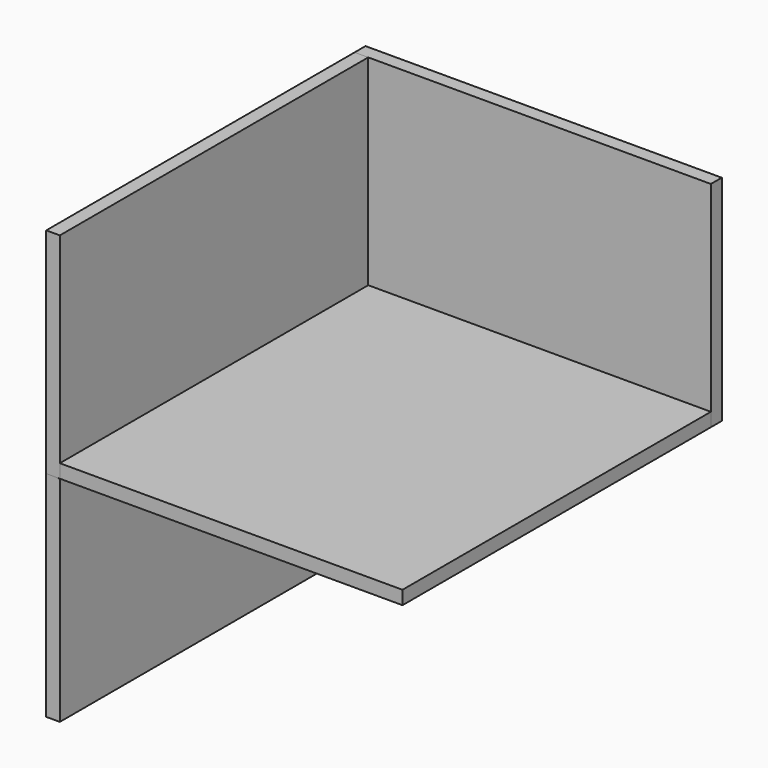
from build123d import *

# Parameters (mm, degrees)
F0_W           = 83.175
F0_H           = 50
F1_DEPTH       = 3.175
F2_W           = 3.175
F2_H           = 50
F3_DEPTH       = 90
F4_W           = 3.175
F4_H           = 50
F5_DEPTH       = 80
F6_W           = 80
F6_H           = 3.175
F7_DEPTH       = 90
F8_W           = 80
F8_H           = 3.175
F9_DEPTH       = 80
F10_W          = 3.175
F10_H          = 50
F11_DEPTH      = 90
F11_DEPTH_BACK = 3.175
F12_R          = 2.5
F13_DEPTH      = 3.175


# Not quite as in the source:
# - a length typed as a fraction of an inch, garbled in the dataset ("3 / 203.2 mm" for 3/8 in), is restored
# - a feature names something its author has since deleted; it is built from what else it names


with BuildPart() as f1:
    # F0 (on Front) → F1 (new body)
    with BuildSketch(Plane.XZ):
        Rectangle(F0_W, F0_H)
    extrude(amount=-F1_DEPTH)


with BuildPart() as f3:
    # F2 (on Front) → F3 (new body)
    with BuildSketch(Plane.XZ):
        with Locations((-40, 0)):
            Rectangle(F2_W, F2_H)
    extrude(amount=F3_DEPTH)


with BuildPart() as f5:
    # F4 (on Front) → F5 (new body)
    with BuildSketch(Plane.XZ):
        with Locations((40, 0)):
            Rectangle(F4_W, F4_H)
    extrude(amount=F5_DEPTH)

    # F12 (on face) → F13 (cut, through all)
    with BuildSketch(Plane.YZ.offset(41.5875)):
        with Locations((-40, -15)):
            Circle(F12_R)
    extrude(amount=-F13_DEPTH, mode=Mode.SUBTRACT)


with BuildPart() as f7:
    # F6 (on Front) → F7 (new body)
    with BuildSketch(Plane.XZ):
        with Locations((1.5875, -23.4125)):
            Rectangle(F6_W, F6_H)
    extrude(amount=F7_DEPTH)


with BuildPart() as f9:
    # F8 (on Front) → F9 (new body)
    with BuildSketch(Plane.XZ):
        with Locations((1.5875, 23.4125)):
            Rectangle(F8_W, F8_H)
    extrude(amount=F9_DEPTH)


with BuildPart() as f11:
    # F10 (on Front) → F11 (new body, two sides)
    with BuildSketch(Plane.XZ) as f11_sk:
        with Locations((-40, -50)):
            Rectangle(F10_W, F10_H)
    extrude(amount=F11_DEPTH)
    extrude(f11_sk.sketch, amount=-F11_DEPTH_BACK)


solid = Compound([f1.part, f3.part, f7.part, f11.part])
